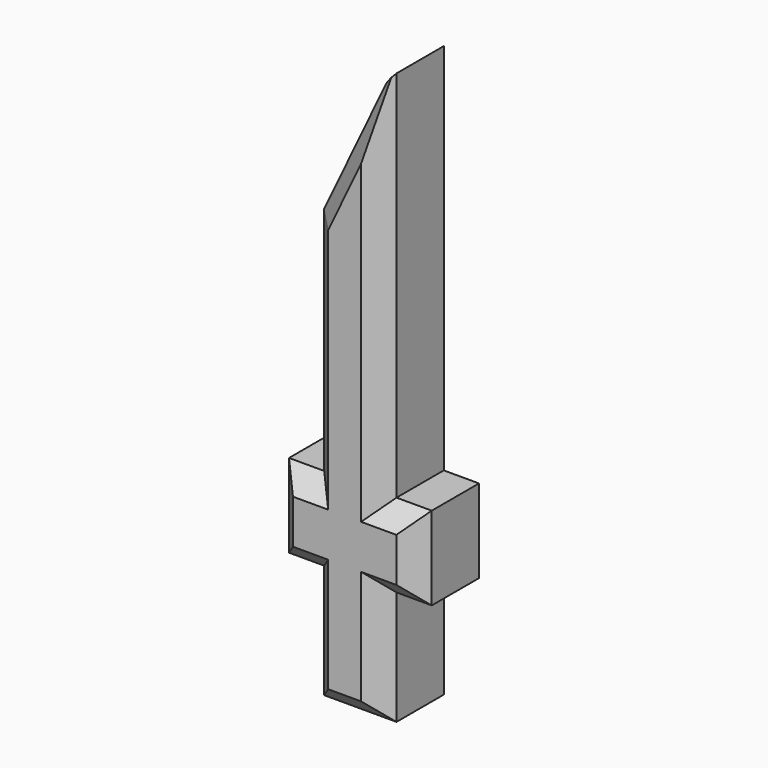
from build123d import *

# Parameters (mm, degrees)
F0_W        = 9.0893283486
F0_H        = 21.5273555368
F0_W_2      = 9.3285199255
F0_H_2      = 29.4207185507
F1_DEPTH    = 25.4
F2_R        = 9.5587418967
F3_DEPTH    = 25.4
F4_C1_SIZE  = 5.08
F4_C2_SIZE  = 5.08
F4_C3_SIZE  = 5.08
F4_C4_SIZE  = 5.08
F4_C5_SIZE  = 5.08
F4_C6_SIZE  = 5.0799
F4_C7_SIZE  = 5.08
F4_C8_SIZE  = 5.08
F4_C9_SIZE  = 5.08
F4_C10_SIZE = 5.08
F4_C11_SIZE = 5.08
F4_C12_SIZE = 5.08
F5_C1_SIZE  = 5.08
F5_C2_SIZE  = 5.08
F5_C3_SIZE  = 5.08
F5_C4_SIZE  = 5.08
F5_C5_SIZE  = 5.08
F5_C6_SIZE  = 5.08
F5_C7_SIZE  = 5.08
F5_C8_SIZE  = 5.08
F5_C9_SIZE  = 5.08
F5_C10_SIZE = 5.08
F5_C11_SIZE = 5.0799
F5_C12_SIZE = 5.08


# Not quite as in the source:
# - a fillet or chamfer is up to 0.001 mm smaller than in the source, because OpenCascade refuses the exact size


with BuildPart() as f1:
    # F0 (on Front) → F1 (new body)
    with BuildSketch(Plane.XZ):
        with Locations((-13.8731840998, -35.7593270019)):
            Rectangle(F0_W, F0_H)
        Polygon((-9.3285199255, -24.9956492335), (-9.3285199255, -46.5230047703), (0, -46.5230047703), (9.3285199255, -46.5230047703), (9.3285199255, -24.9956492335), (9.3285199255, 34.5633625984), (9.3285199255, 71.3990554214), (6.6973981448, 68.2895556092), (-9.3285199255, 34.5633625984), align=None)
        with Locations((13.8731840998, -35.7593270019)):
            Rectangle(F0_W, F0_H)
        with Locations((-4.6642599627, -61.2333640456)):
            Rectangle(F0_W_2, F0_H_2)
        with Locations((4.6642599627, -61.2333640456)):
            Rectangle(F0_W_2, F0_H_2)
    extrude(amount=F1_DEPTH)

    # F2 (on Front) → F3 (join)
    with BuildSketch(Plane.XZ):
        with Locations((0, -37.1944867074)):
            Circle(F2_R)
    extrude(amount=F3_DEPTH)

    # F4: chamfer of 5.08 on 13 edges, made by hand

    # F4_c1
    f4_c1_edges = [f1.edges().sort_by_distance(p)[0] for p in [
        (-13.8731840998, 0, -46.5230047703),
    ]]
    chamfer(f4_c1_edges, length=F4_C1_SIZE)

    # F4_c2
    f4_c2_edges = [f1.edges().sort_by_distance(p)[0] for p in [
        (-18.4178482741, 0, -33.2193270019),
    ]]
    chamfer(f4_c2_edges, length=F4_C2_SIZE)

    # F4_c3
    f4_c3_edges = [f1.edges().sort_by_distance(p)[0] for p in [
        (-9.3285199255, 0, -61.2333640456),
    ]]
    chamfer(f4_c3_edges, length=F4_C3_SIZE)

    # F4_c4
    f4_c4_edges = [f1.edges().sort_by_distance(p)[0] for p in [
        (2.54, 0, -75.943723321),
    ]]
    chamfer(f4_c4_edges, length=F4_C4_SIZE)

    # F4_c5
    f4_c5_edges = [f1.edges().sort_by_distance(p)[0] for p in [
        (9.3285199255, 0, -58.6933640456),
    ]]
    chamfer(f4_c5_edges, length=F4_C5_SIZE)

    # F4_c6 (size 5.08 in the source; OpenCascade refuses exactly that, so slightly less here)
    f4_c6_edges = [f1.edges().sort_by_distance(p)[0] for p in [
        (13.8731840998, 0, -46.5230047703),
    ]]
    chamfer(f4_c6_edges, length=F4_C6_SIZE)

    # F4_c7
    f4_c7_edges = [f1.edges().sort_by_distance(p)[0] for p in [
        (18.4178482741, 0, -33.2193770019),
    ]]
    chamfer(f4_c7_edges, length=F4_C7_SIZE)

    # F4_c8
    f4_c8_edges = [f1.edges().sort_by_distance(p)[0] for p in [
        (11.3331840998, 0, -24.9956492335),
    ]]
    chamfer(f4_c8_edges, length=F4_C8_SIZE)

    # F4_c9
    f4_c9_edges = [f1.edges().sort_by_distance(p)[0] for p in [
        (9.3285199255, 0, 23.2017030939),
    ]]
    chamfer(f4_c9_edges, length=F4_C9_SIZE)

    # F4_c10
    f4_c10_edges = [f1.edges().sort_by_distance(p)[0] for p in [
        (-2.54, 0, 48.8496538587),
    ]]
    chamfer(f4_c10_edges, length=F4_C10_SIZE)

    # F4_c11
    f4_c11_edges = [f1.edges().sort_by_distance(p)[0] for p in [
        (-9.3285199255, 0, -1.1343040268),
    ]]
    chamfer(f4_c11_edges, length=F4_C11_SIZE)

    # F4_c12
    f4_c12_edges = [f1.edges().sort_by_distance(p)[0] for p in [
        (-11.3331840998, 0, -24.9956492335),
    ]]
    chamfer(f4_c12_edges, length=F4_C12_SIZE)

    # F5: chamfer of 5.08 on 13 edges, made by hand

    # F5_c1
    f5_c1_edges = [f1.edges().sort_by_distance(p)[0] for p in [
        (-18.4178482741, -25.4, -35.7593270019),
    ]]
    chamfer(f5_c1_edges, length=F5_C1_SIZE)

    # F5_c2
    f5_c2_edges = [f1.edges().sort_by_distance(p)[0] for p in [
        (-11.3331840998, -25.4, -24.9956492335),
    ]]
    chamfer(f5_c2_edges, length=F5_C2_SIZE)

    # F5_c3
    f5_c3_edges = [f1.edges().sort_by_distance(p)[0] for p in [
        (-11.3331840998, -25.4, -46.5230047703),
    ]]
    chamfer(f5_c3_edges, length=F5_C3_SIZE)

    # F5_c4
    f5_c4_edges = [f1.edges().sort_by_distance(p)[0] for p in [
        (-9.3285199255, -25.4, 4.7838566825),
    ]]
    chamfer(f5_c4_edges, length=F5_C4_SIZE)

    # F5_c5
    f5_c5_edges = [f1.edges().sort_by_distance(p)[0] for p in [
        (-9.3285199255, -25.4, -61.2333640456),
    ]]
    chamfer(f5_c5_edges, length=F5_C5_SIZE)

    # F5_c6
    f5_c6_edges = [f1.edges().sort_by_distance(p)[0] for p in [
        (1.2244391096, -25.4, 56.7718333827),
    ]]
    chamfer(f5_c6_edges, length=F5_C6_SIZE)

    # F5_c7
    f5_c7_edges = [f1.edges().sort_by_distance(p)[0] for p in [
        (2.54, -25.4, -75.943723321),
    ]]
    chamfer(f5_c7_edges, length=F5_C7_SIZE)

    # F5_c8
    f5_c8_edges = [f1.edges().sort_by_distance(p)[0] for p in [
        (9.3285199255, -25.4, 18.4973615123),
    ]]
    chamfer(f5_c8_edges, length=F5_C8_SIZE)

    # F5_c9
    f5_c9_edges = [f1.edges().sort_by_distance(p)[0] for p in [
        (13.8731840998, -25.4, -46.5230047703),
    ]]
    chamfer(f5_c9_edges, length=F5_C9_SIZE)

    # F5_c10
    f5_c10_edges = [f1.edges().sort_by_distance(p)[0] for p in [
        (9.3285199255, -25.4, -58.6933640456),
    ]]
    chamfer(f5_c10_edges, length=F5_C10_SIZE)

    # F5_c11 (size 5.08 in the source; OpenCascade refuses exactly that, so slightly less here)
    f5_c11_edges = [f1.edges().sort_by_distance(p)[0] for p in [
        (13.8731840998, -25.4, -24.9956492335),
    ]]
    chamfer(f5_c11_edges, length=F5_C11_SIZE)

    # F5_c12
    f5_c12_edges = [f1.edges().sort_by_distance(p)[0] for p in [
        (18.4178482741, -25.4, -35.7592770019),
    ]]
    chamfer(f5_c12_edges, length=F5_C12_SIZE)


solid = f1.part
